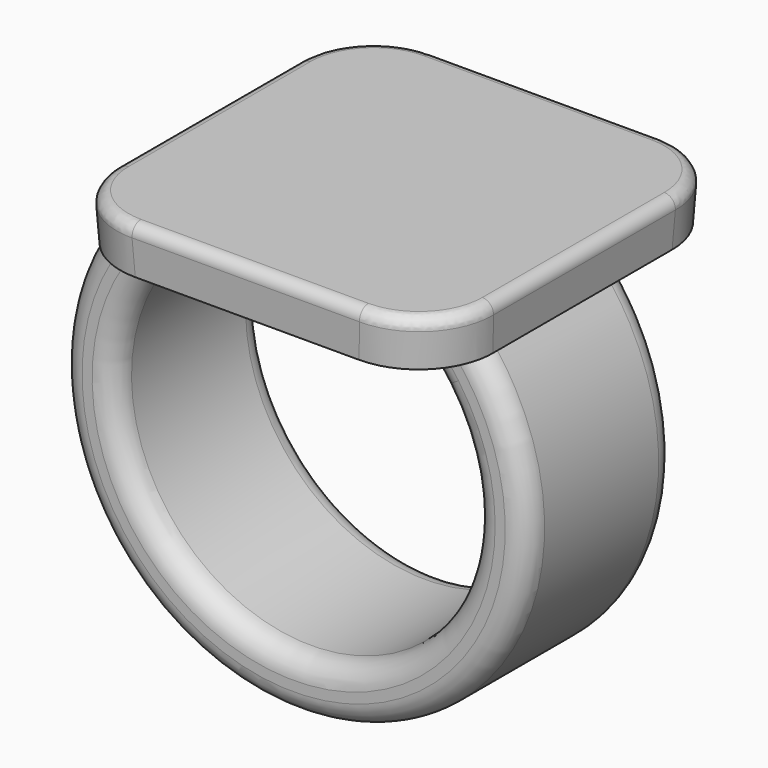
from build123d import *

# Parameters (mm, degrees)
F0_W                   = 25.4
F0_H                   = 25.4
F1_DEPTH               = 3.175
DRAFT_F1_DRAFTED_ANGLE = -3
F3_W                   = 5.08
F3_H                   = 12.7
F6_DEPTH               = 8.7411567288
F6_DEPTH_BACK          = 3.9588432712
F7_T4_DEPTH            = 28.5142315252
F7_T10_DEPTH           = 28.5142315252
F7_T16_DEPTH           = 28.5142315252
F7_T22_DEPTH           = 28.5142315252
F8_T4_ANGLE            = 284.5817422952
F8_T9_ANGLE            = 34.2022068088
F8_T14_ANGLE           = 284.5817422952
F8_T19_ANGLE           = 34.2022068088
F8_T24_ANGLE           = 281.6460775509
F8_T29_ANGLE           = 281.6460775509
F9_R                   = 0.762


# Not quite as in the source:
# - a fillet or chamfer that OpenCascade refuses, or shapes differently, is made with other operations: its cross-section is extruded or revolved along the edge and cut away or added
# - an extrude with a draft is written as a straight extrude whose walls are then drafted


with BuildPart() as f1:
    # F0 (on Top) → F1 (new body)
    with BuildSketch(Plane.XY):
        Rectangle(F0_W, F0_H)
    extrude(amount=F1_DEPTH)

    # draft_F1_drafted
    draft_f1_drafted_walls = [f1.faces().sort_by_distance(p)[0] for p in [
        (12.7, 0, 2.1166666667),
        (0, 12.7, 2.1166666667),
        (-12.7, 0, 2.1166666667),
        (0, -12.7, 2.1166666667),
    ]]
    draft(draft_f1_drafted_walls, neutral_plane=Plane.XY, angle=DRAFT_F1_DRAFTED_ANGLE)

    # F4: sweep along a path in F2
    with BuildLine(Plane.XZ) as f4_path:
        ThreePointArc((-10.16, 0), (0, -23.5582897328), (10.16, 0))
    # F3 (on face) → F4 (sweep)
    with BuildSketch(Plane(origin=(0, 0, 0), x_dir=(1, 0, 0), z_dir=(0, 0, -1))):
        with Locations((-10.16, 2.3911567288)):
            Rectangle(F3_W, F3_H)
    sweep(path=f4_path.line)

    # F5 (on Front) → F6 (join, two sides)
    with BuildSketch(Plane.XZ) as f6_sk:
        with BuildLine():
            Line((10.0130578512, -2.535746045), (10.16, 0))
            Line((10.16, 0), (7.62, 0))
            ThreePointArc((7.62, 0), (8.9072265211, -1.1822790439), (10.0130578512, -2.535746045))
        make_face()
    extrude(amount=F6_DEPTH)
    extrude(f6_sk.sketch, amount=-F6_DEPTH_BACK)

    # F7: fillet of radius 5.08 on 4 edges, made by hand


with BuildPart() as f7_tool2:
    # F7_s3 → F7_t4 (new body)
    with BuildSketch(Plane(origin=(-0.592560758, 0.592560758, -11.3067328194), x_dir=(0.7071067812, 0.7071067812, 0), z_dir=(0.0522644277, -0.0522644277, 0.9972646886))):
        with BuildLine():
            ThreePointArc((3.5871795969, -14.3340171051), (0, -15.8169985425), (-3.5871795969, -14.3340171051))
            Line((-3.5871795969, -14.3340171051), (-3.6589231888, -14.4059574764))
            Line((-3.6589231888, -14.4059574764), (0, -18.054872371))
            Line((0, -18.054872371), (3.6589231888, -14.4059574764))
            Line((3.6589231888, -14.4059574764), (3.5871795969, -14.3340171051))
        make_face()
    extrude(amount=F7_T4_DEPTH)

    split(bisect_by=Plane.XY, keep=Keep.TOP)

    split(bisect_by=Plane.XY.offset(3.175), keep=Keep.BOTTOM)


with BuildPart() as f1_1:
    add(f1.part)

    # F7_t1: cut F7_tool2
    add(f7_tool2.part, mode=Mode.SUBTRACT)


with BuildPart() as f7_tool8:
    # F7_s9 → F7_t10 (new body)
    with BuildSketch(Plane(origin=(-0.592560758, -0.592560758, -11.3067328194), x_dir=(-0.7071067812, 0.7071067812, 0), z_dir=(0.0522644277, 0.0522644277, 0.9972646886))):
        with BuildLine():
            ThreePointArc((-3.5871795969, -14.3340171051), (0, -15.8169985425), (3.5871795969, -14.3340171051))
            Line((3.5871795969, -14.3340171051), (3.6589231888, -14.4059574764))
            Line((3.6589231888, -14.4059574764), (0, -18.054872371))
            Line((0, -18.054872371), (-3.6589231888, -14.4059574764))
            Line((-3.6589231888, -14.4059574764), (-3.5871795969, -14.3340171051))
        make_face()
    extrude(amount=F7_T10_DEPTH)

    split(bisect_by=Plane.XY, keep=Keep.TOP)

    split(bisect_by=Plane.XY.offset(3.175), keep=Keep.BOTTOM)


with BuildPart() as f1_2:
    add(f1_1.part)

    # F7_t7: cut F7_tool8
    add(f7_tool8.part, mode=Mode.SUBTRACT)


with BuildPart() as f7_tool14:
    # F7_s15 → F7_t16 (new body)
    with BuildSketch(Plane(origin=(0.592560758, -0.592560758, -11.3067328194), x_dir=(-0.7071067812, -0.7071067812, 0), z_dir=(-0.0522644277, 0.0522644277, 0.9972646886))):
        with BuildLine():
            ThreePointArc((3.5871795969, -14.3340171051), (0, -15.8169985425), (-3.5871795969, -14.3340171051))
            Line((-3.5871795969, -14.3340171051), (-3.6589231888, -14.4059574764))
            Line((-3.6589231888, -14.4059574764), (0, -18.054872371))
            Line((0, -18.054872371), (3.6589231888, -14.4059574764))
            Line((3.6589231888, -14.4059574764), (3.5871795969, -14.3340171051))
        make_face()
    extrude(amount=F7_T16_DEPTH)

    split(bisect_by=Plane.XY.offset(3.175), keep=Keep.BOTTOM)

    split(bisect_by=Plane.XY, keep=Keep.TOP)


with BuildPart() as f1_3:
    add(f1_2.part)

    # F7_t13: cut F7_tool14
    add(f7_tool14.part, mode=Mode.SUBTRACT)


with BuildPart() as f7_tool20:
    # F7_s21 → F7_t22 (new body)
    with BuildSketch(Plane(origin=(0.592560758, 0.592560758, -11.3067328194), x_dir=(0.7071067812, -0.7071067812, 0), z_dir=(-0.0522644277, -0.0522644277, 0.9972646886))):
        with BuildLine():
            ThreePointArc((-3.5871795969, -14.3340171051), (0, -15.8169985425), (3.5871795969, -14.3340171051))
            Line((3.5871795969, -14.3340171051), (3.6589231888, -14.4059574764))
            Line((3.6589231888, -14.4059574764), (0, -18.054872371))
            Line((0, -18.054872371), (-3.6589231888, -14.4059574764))
            Line((-3.6589231888, -14.4059574764), (-3.5871795969, -14.3340171051))
        make_face()
    extrude(amount=F7_T22_DEPTH)

    split(bisect_by=Plane.XY.offset(3.175), keep=Keep.BOTTOM)

    split(bisect_by=Plane.XY, keep=Keep.TOP)


with BuildPart() as f1_4:
    add(f1_3.part)

    # F7_t19: cut F7_tool20
    add(f7_tool20.part, mode=Mode.SUBTRACT)

    # F8: fillet of radius 1.524 on 6 edges, made by hand


with BuildPart() as f8_tool2:
    # F8_s3 → F8_t4 (revolve)
    with BuildSketch(Plane(origin=(-3.1549079732, 0, -1.1843830071), x_dir=(0, 1, 0), z_dir=(0.9362030192, 0, 0.3514596802))):
        with BuildLine():
            ThreePointArc((-8.7415567288, 4.7958163548), (-8.2947874634, 3.7172199348), (-7.2161910434, 3.2704506693))
            Line((-7.2161910434, 3.2704506693), (-7.2161910434, 3.1179141008))
            ThreePointArc((-7.2161910434, 3.1179141008), (-7.9786738861, 3.1183141008), (-8.7411567288, 3.1183141008))
            Line((-8.7411567288, 3.1183141008), (-8.8936932974, 3.2708506693))
            ThreePointArc((-8.8936932974, 3.2708506693), (-8.8936932974, 4.0333335121), (-8.8940932974, 4.7958163548))
            Line((-8.8940932974, 4.7958163548), (-8.7415567288, 4.7958163548))
        make_face()
    revolve(axis=Axis((0, -8.7411567288, -9.5882897328), (0, -1, 0)), revolution_arc=F8_T4_ANGLE)

    split(bisect_by=Plane.XY, keep=Keep.BOTTOM)


with BuildPart() as f1_5:
    add(f1_4.part)

    # F8_t1: cut F8_tool2
    add(f8_tool2.part, mode=Mode.SUBTRACT)


with BuildPart() as f8_tool7:
    # F8_s8 → F8_t9 (revolve)
    with BuildSketch(Plane(origin=(3.1628144119, 0, -1.1913084844), x_dir=(0, 1, 0), z_dir=(-0.9358171874, 0, 0.3524857326))):
        with BuildLine():
            ThreePointArc((-8.7415567288, -4.7995158219), (-8.2947874634, -3.720919402), (-7.2161910434, -3.2741501365))
            Line((-7.2161910434, -3.2741501365), (-7.2161910434, -3.1216135679))
            ThreePointArc((-7.2161910434, -3.1216135679), (-7.9786738861, -3.1220135679), (-8.7411567288, -3.1220135679))
            Line((-8.7411567288, -3.1220135679), (-8.8936932974, -3.2745501365))
            ThreePointArc((-8.8936932974, -3.2745501365), (-8.8936932974, -4.0370329792), (-8.8940932974, -4.7995158219))
            Line((-8.8940932974, -4.7995158219), (-8.7415567288, -4.7995158219))
        make_face()
    revolve(axis=Axis((0, -8.7411567288, -9.5882897328), (0, 1, 0)), revolution_arc=F8_T9_ANGLE)

    split(bisect_by=Plane.XY, keep=Keep.BOTTOM)


with BuildPart() as f1_6:
    add(f1_5.part)

    # F8_t6: cut F8_tool7
    add(f8_tool7.part, mode=Mode.SUBTRACT)


with BuildPart() as f8_tool12:
    # F8_s13 → F8_t14 (revolve)
    with BuildSketch(Plane(origin=(-3.1549079732, 0, -1.1843830071), x_dir=(0, 1, 0), z_dir=(0.9362030192, 0, 0.3514596802))):
        with BuildLine():
            ThreePointArc((3.9592432712, 4.7958163548), (3.5124740057, 3.7172199348), (2.4338775857, 3.2704506693))
            Line((2.4338775857, 3.2704506693), (2.4338775857, 3.1179141008))
            ThreePointArc((2.4338775857, 3.1179141008), (3.1963604284, 3.1183141008), (3.9588432712, 3.1183141008))
            Line((3.9588432712, 3.1183141008), (4.1113798397, 3.2708506693))
            ThreePointArc((4.1113798397, 3.2708506693), (4.1113798397, 4.0333335121), (4.1117798397, 4.7958163548))
            Line((4.1117798397, 4.7958163548), (3.9592432712, 4.7958163548))
        make_face()
    revolve(axis=Axis((0, 3.9588432712, -9.5882897328), (0, -1, 0)), revolution_arc=F8_T14_ANGLE)

    split(bisect_by=Plane.XY, keep=Keep.BOTTOM)


with BuildPart() as f1_7:
    add(f1_6.part)

    # F8_t11: cut F8_tool12
    add(f8_tool12.part, mode=Mode.SUBTRACT)


with BuildPart() as f8_tool17:
    # F8_s18 → F8_t19 (revolve)
    with BuildSketch(Plane(origin=(3.1628144119, 0, -1.1913084844), x_dir=(0, 1, 0), z_dir=(-0.9358171874, 0, 0.3524857326))):
        with BuildLine():
            ThreePointArc((3.9592432712, -4.7995158219), (3.5124740057, -3.720919402), (2.4338775857, -3.2741501365))
            Line((2.4338775857, -3.2741501365), (2.4338775857, -3.1216135679))
            ThreePointArc((2.4338775857, -3.1216135679), (3.1963604284, -3.1220135679), (3.9588432712, -3.1220135679))
            Line((3.9588432712, -3.1220135679), (4.1113798397, -3.2745501365))
            ThreePointArc((4.1113798397, -3.2745501365), (4.1113798397, -4.0370329792), (4.1117798397, -4.7995158219))
            Line((4.1117798397, -4.7995158219), (3.9592432712, -4.7995158219))
        make_face()
    revolve(axis=Axis((0, 3.9588432712, -9.5882897328), (0, 1, 0)), revolution_arc=F8_T19_ANGLE)

    split(bisect_by=Plane.XY, keep=Keep.BOTTOM)


with BuildPart() as f1_8:
    add(f1_7.part)

    # F8_t16: cut F8_tool17
    add(f8_tool17.part, mode=Mode.SUBTRACT)


with BuildPart() as f8_tool22:
    # F8_s23 → F8_t24 (revolve)
    with BuildSketch(Plane(origin=(-4.6954488846, 0, -3.8263717671), x_dir=(0, 1, 0), z_dir=(0.7751985666, 0, 0.6317176445))):
        with BuildLine():
            ThreePointArc((2.4338775857, 8.4806259324), (3.5124740057, 8.0338566669), (3.9592432712, 6.9552602469))
            Line((3.9592432712, 6.9552602469), (4.1117798397, 6.9552602469))
            ThreePointArc((4.1117798397, 6.9552602469), (4.1113798397, 7.7177430897), (4.1113798397, 8.4802259324))
            Line((4.1113798397, 8.4802259324), (3.9588432712, 8.6327625009))
            ThreePointArc((3.9588432712, 8.6327625009), (3.1963604284, 8.6327625009), (2.4338775857, 8.6331625009))
            Line((2.4338775857, 8.6331625009), (2.4338775857, 8.4806259324))
        make_face()
    revolve(axis=Axis((0, 3.9588432712, -9.5882897328), (0, -1, 0)), revolution_arc=F8_T24_ANGLE)

    split(bisect_by=Plane.XY, keep=Keep.BOTTOM)


with BuildPart() as f1_9:
    add(f1_8.part)

    # F8_t21: cut F8_tool22
    add(f8_tool22.part, mode=Mode.SUBTRACT)


with BuildPart() as f8_tool27:
    # F8_s28 → F8_t29 (revolve)
    with BuildSketch(Plane(origin=(-4.6954488846, 0, -3.8263717671), x_dir=(0, 1, 0), z_dir=(0.7751985666, 0, 0.6317176445))):
        with BuildLine():
            ThreePointArc((-7.2161910434, 8.4806259324), (-8.2947874634, 8.0338566669), (-8.7415567288, 6.9552602469))
            Line((-8.7415567288, 6.9552602469), (-8.8940932974, 6.9552602469))
            ThreePointArc((-8.8940932974, 6.9552602469), (-8.8936932974, 7.7177430897), (-8.8936932974, 8.4802259324))
            Line((-8.8936932974, 8.4802259324), (-8.7411567288, 8.6327625009))
            ThreePointArc((-8.7411567288, 8.6327625009), (-7.9786738861, 8.6327625009), (-7.2161910434, 8.6331625009))
            Line((-7.2161910434, 8.6331625009), (-7.2161910434, 8.4806259324))
        make_face()
    revolve(axis=Axis((0, -8.7411567288, -9.5882897328), (0, -1, 0)), revolution_arc=F8_T29_ANGLE)

    split(bisect_by=Plane.XY, keep=Keep.BOTTOM)


with BuildPart() as f1_10:
    add(f1_9.part)

    # F8_t26: cut F8_tool27
    add(f8_tool27.part, mode=Mode.SUBTRACT)

    # F9
    f9_edges = [f1_10.edges().sort_by_distance(p)[0] for p in [
        (-11.381378, 11.381378, 3.175),
        (0, 12.866395, 3.175),
        (11.381378, 11.381378, 3.175),
        (12.866395, 0, 3.175),
        (11.381378, -11.381378, 3.175),
        (0, -12.866395, 3.175),
        (-11.381378, -11.381378, 3.175),
        (-12.866395, 0, 3.175),
    ]]
    fillet(f9_edges, radius=F9_R)


solid = f1_10.part
